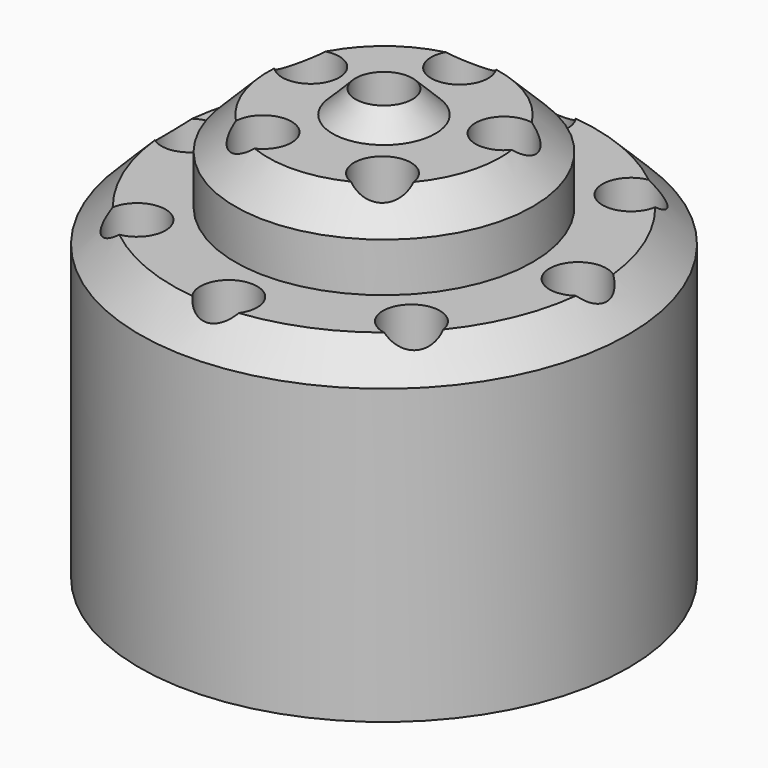
from build123d import *

# Parameters (mm, degrees)
F0_R     = 38.1
F0_R_2   = 4.445
F0_R_3   = 23.1824441608
F1_DEPTH = 50.8
F0_R_4   = 8.0064033383
F2_DEPTH = 63.5
F3_DEPTH = 68.58
F4_DEPTH = 2.54
F5_DEPTH = 25.4
F6_DEPTH = 38.1


# Not quite as in the source:
# - a fillet or chamfer that OpenCascade refuses, or shapes differently, is made with other operations: its cross-section is extruded or revolved along the edge and cut away or added


with BuildPart() as f1:
    # F0 (on Top) → F1 (new body)
    with BuildSketch(Plane.XY):
        Circle(F0_R)
        with Locations((-21.3879767226, -21.3879767226)):
            Circle(F0_R_2, mode=Mode.SUBTRACT)
        with Locations((0, -30.2471667528)):
            Circle(F0_R_2, mode=Mode.SUBTRACT)
        with Locations((21.3879767226, -21.3879767226)):
            Circle(F0_R_2, mode=Mode.SUBTRACT)
        with Locations((-30.2471667528, 0)):
            Circle(F0_R_2, mode=Mode.SUBTRACT)
        with Locations((-21.3879767226, 21.3879767226)):
            Circle(F0_R_2, mode=Mode.SUBTRACT)
        Circle(F0_R_3, mode=Mode.SUBTRACT)
        with Locations((30.2471667528, 0)):
            Circle(F0_R_2, mode=Mode.SUBTRACT)
        with Locations((0, 30.2471667528)):
            Circle(F0_R_2, mode=Mode.SUBTRACT)
        with Locations((21.3879767226, 21.3879767226)):
            Circle(F0_R_2, mode=Mode.SUBTRACT)
    extrude(amount=F1_DEPTH)

    # F0 (on Top) → F2 (join)
    with BuildSketch(Plane.XY):
        Circle(F0_R_3)
        with Locations((-8.6240968668, -12.7810694279)):
            Circle(F0_R_2, mode=Mode.SUBTRACT)
        with Locations((9.4905268716, -12.1515711819)):
            Circle(F0_R_2, mode=Mode.SUBTRACT)
        with Locations((-14.8205118576, 4.2524358628)):
            Circle(F0_R_2, mode=Mode.SUBTRACT)
        with Locations((-0.5354831918, 15.4092193261)):
            Circle(F0_R_2, mode=Mode.SUBTRACT)
        Circle(F0_R_4, mode=Mode.SUBTRACT)
        with Locations((14.4895650446, 5.2709854208)):
            Circle(F0_R_2, mode=Mode.SUBTRACT)
    extrude(amount=F2_DEPTH)

    # F0 (on Top) → F3 (join)
    with BuildSketch(Plane.XY):
        Circle(F0_R_4)
        Circle(F0_R_2, mode=Mode.SUBTRACT)
    extrude(amount=F3_DEPTH)

    # F0 (on Top) → F4 (join)
    with BuildSketch(Plane.XY):
        with Locations((-30.2471667528, 0)):
            Circle(F0_R_2)
        with Locations((-21.3879767226, -21.3879767226)):
            Circle(F0_R_2)
        with Locations((0, -30.2471667528)):
            Circle(F0_R_2)
        with Locations((21.3879767226, -21.3879767226)):
            Circle(F0_R_2)
        with Locations((21.3879767226, 21.3879767226)):
            Circle(F0_R_2)
        with Locations((0, 30.2471667528)):
            Circle(F0_R_2)
        with Locations((-21.3879767226, 21.3879767226)):
            Circle(F0_R_2)
        with Locations((30.2471667528, 0)):
            Circle(F0_R_2)
    extrude(amount=F4_DEPTH)

    # F0 (on Top) → F5 (join)
    with BuildSketch(Plane.XY):
        with Locations((-8.6240968668, -12.7810694279)):
            Circle(F0_R_2)
        with Locations((9.4905268716, -12.1515711819)):
            Circle(F0_R_2)
        with Locations((14.4895650446, 5.2709854208)):
            Circle(F0_R_2)
        with Locations((-0.5354831918, 15.4092193261)):
            Circle(F0_R_2)
        with Locations((-14.8205118576, 4.2524358628)):
            Circle(F0_R_2)
    extrude(amount=F5_DEPTH)

    # F0 (on Top) → F6 (join)
    with BuildSketch(Plane.XY):
        Circle(F0_R_2)
    extrude(amount=F6_DEPTH)

    # F7: chamfer of 5.08 on 3 edges, made by hand

    # F7_s1 → F7_t2 (revolve, cut)
    with BuildSketch(Plane.XZ):
        Polygon((38.1, 45.72), (33.02, 50.8), (38.1, 50.8), align=None)
    revolve(axis=Axis((0, 0, 50.8), (0, 0, 1)), mode=Mode.SUBTRACT)

    # F7_s3 → F7_t4 (revolve, cut)
    with BuildSketch(Plane.XZ):
        Polygon((23.1824441608, 58.42), (18.1024441608, 63.5), (23.1824441608, 63.5), align=None)
    revolve(axis=Axis((0, 0, 63.5), (0, 0, 1)), mode=Mode.SUBTRACT)


with BuildPart() as f7_tool6:
    # F7_s7 → F7_t8 (revolve)
    with BuildSketch(Plane.XZ):
        Polygon((8.0064033383, 63.5), (2.9264033383, 68.58), (8.0064033383, 68.58), align=None)
    revolve(axis=Axis((0, 0, 68.58), (0, 0, 1)))

    split(bisect_by=Plane.XY.offset(63.5), keep=Keep.TOP)


with BuildPart() as f1_1:
    add(f1.part)

    # F7_t5: cut F7_tool6
    add(f7_tool6.part, mode=Mode.SUBTRACT)


solid = f1_1.part
